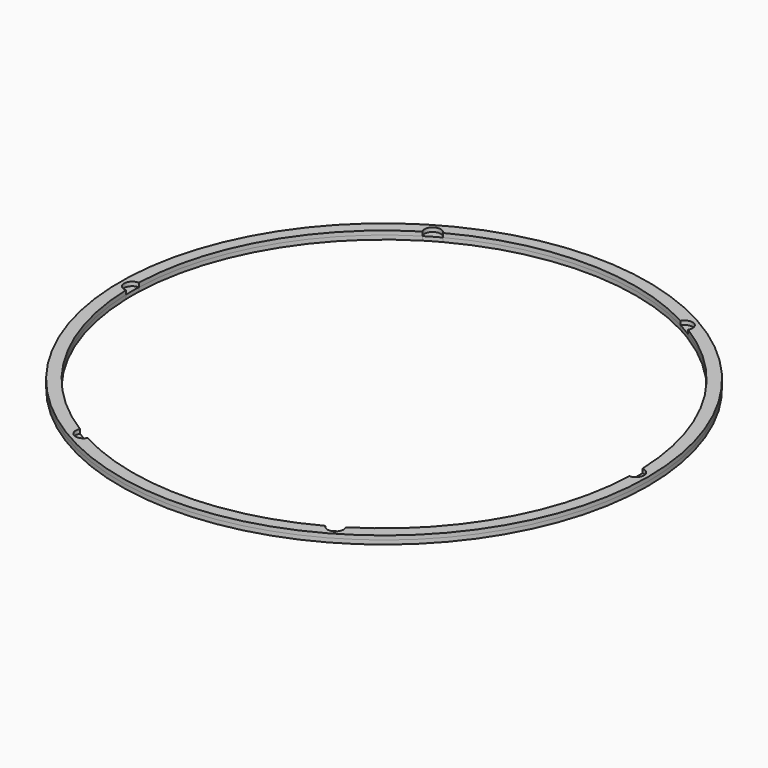
from build123d import *
from build123d import SkipClean  # not in build123d's __all__

# Parameters (mm, degrees)
F0_R     = 65.5
F1_DEPTH = 2
F2_R     = 65.5
F2_R_2   = 62.5
F3_DEPTH = 1


with BuildPart() as f1:
    # F0 (on Top) → F1 (new body)
    with BuildSketch(Plane.XY):
        Circle(F0_R)
        with BuildLine():
            ThreePointArc((32.9658290909, 53.0990029318), (54.1265877365, 31.25), (62.468, 1.9997439836))
            ThreePointArc((62.468, 1.9997439836), (64.5, 0), (62.468, -1.9997439836))
            ThreePointArc((62.468, -1.9997439836), (54.1265877365, -31.25), (32.9658290909, -53.0990029318))
            ThreePointArc((32.9658290909, -53.0990029318), (32.25, -55.8586385441), (29.5021709091, -55.0987469154))
            ThreePointArc((29.5021709091, -55.0987469154), (0, -62.5), (-29.5021709091, -55.0987469154))
            ThreePointArc((-29.5021709091, -55.0987469154), (-32.25, -55.8586385441), (-32.9658290909, -53.0990029318))
            ThreePointArc((-32.9658290909, -53.0990029318), (-54.1265877365, -31.25), (-62.468, -1.9997439836))
            ThreePointArc((-62.468, -1.9997439836), (-64.5, 0), (-62.468, 1.9997439836))
            ThreePointArc((-62.468, 1.9997439836), (-54.1265877365, 31.25), (-32.9658290909, 53.0990029318))
            ThreePointArc((-32.9658290909, 53.0990029318), (-32.25, 55.8586385441), (-29.5021709091, 55.0987469154))
            ThreePointArc((-29.5021709091, 55.0987469154), (0, 62.5), (29.5021709091, 55.0987469154))
            ThreePointArc((29.5021709091, 55.0987469154), (32.25, 55.8586385441), (32.9658290909, 53.0990029318))
        make_face(mode=Mode.SUBTRACT)
    extrude(amount=F1_DEPTH)

    # F2 (on Top) → F3 (join)
    with BuildSketch(Plane.XY):
        Circle(F2_R)
        Circle(F2_R_2, mode=Mode.SUBTRACT)
    with SkipClean():  # cleaning this boolean's faces spoils the solid; the shape is the same uncleaned
        extrude(amount=F3_DEPTH)


solid = f1.part
